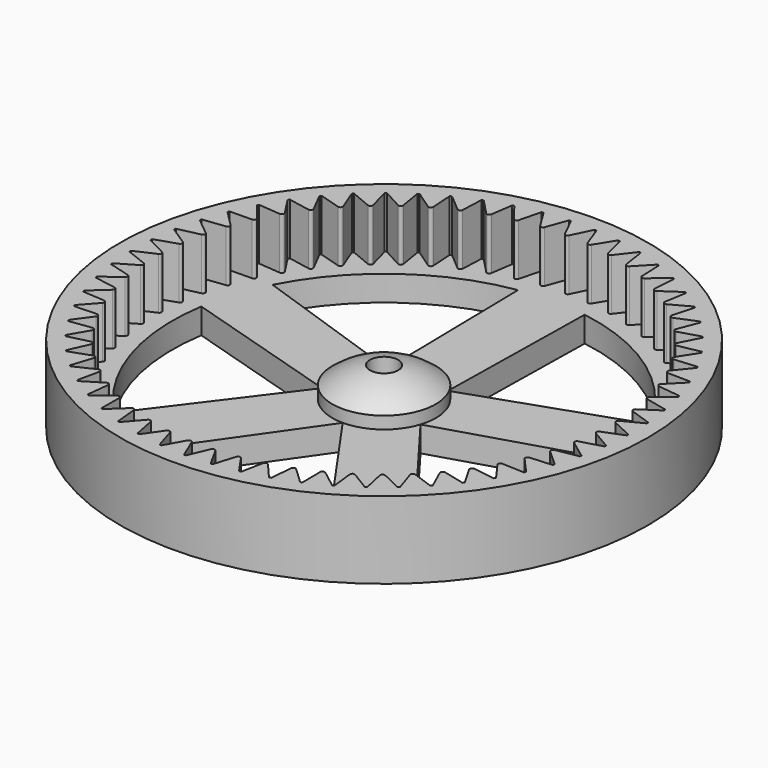
from build123d import *

# Parameters (mm, degrees)
F0_R            = 28.05
F1_DEPTH        = 2.7
F3_DEPTH        = 5.5
F3_COPIES_COUNT = 61
F2_R            = 28.05
F4_DEPTH        = 5.5
F8_DEPTH        = 2.7
F8_COPIES_COUNT = 5
F7_R            = 1.5
F9_DEPTH        = 1.5
F10_DEPTH       = 8.201


# Not quite as in the source:
# - a pattern or mirror of a feature is missing from the dataset's text; its kind, count and spacing are read off the source's solid
# - a feature names something its author has since deleted; it is built from what else it names


with BuildPart() as f1:
    # F0 (on Top) → F1 (new body)
    with BuildSketch(Plane.XY):
        Circle(F0_R)
    extrude(amount=F1_DEPTH)

    # F2 (on face) → F3 (join)
    with BuildSketch(Plane.XY.offset(2.7)):
        with BuildLine():
            ThreePointArc((-1.2632800726, 26.4198149777), (0, 26.45), (1.2632800726, 26.4198149777))
            Line((1.2632800726, 26.4198149777), (1.2934127659, 27.05))
            Line((1.2934127659, 27.05), (-1.2934127659, 27.05))
            Line((-1.2934127659, 27.05), (-1.2632800726, 26.4198149777))
        make_face()
        with BuildLine():
            Line((0.2246985116, 24.2904072133), (1.2632800726, 26.4198149777))
            ThreePointArc((1.2632800726, 26.4198149777), (0, 26.45), (-1.2632800726, 26.4198149777))
            Line((-1.2632800726, 26.4198149777), (-0.2246985116, 24.2904072133))
            ThreePointArc((-0.2246985116, 24.2904072133), (0, 24.15), (0.2246985116, 24.2904072133))
        make_face()
    f3 = extrude(amount=F3_DEPTH)

    # F3_copies: F3 ×61 about axis
    f3_copies_axis = Axis((0, 0, 0), (0, 0, 1))
    for i in range(1, F3_COPIES_COUNT):
        add(f3.rotate(f3_copies_axis, i * 360 / F3_COPIES_COUNT))

    # F2 (on face) → F4 (join, through all)
    with BuildSketch(Plane.XY.offset(2.7)):
        Circle(F2_R)
        with BuildLine():
            ThreePointArc((1.2632800726, 26.4198149777), (19.1444020267, 18.2508731583), (26.45, 0))
            ThreePointArc((26.45, 0), (-18.2508731583, -19.1444020267), (-1.2632800726, 26.4198149777))
            Line((-1.2632800726, 26.4198149777), (-1.2934127659, 27.05))
            Line((-1.2934127659, 27.05), (1.2934127659, 27.05))
            Line((1.2934127659, 27.05), (1.2632800726, 26.4198149777))
        make_face(mode=Mode.SUBTRACT)
    extrude(amount=F4_DEPTH)

    # F5 (on Front) → F6 (revolve)
    with BuildSketch(Plane.XZ):
        with BuildLine():
            Line((-5.5, 4), (-5.5, 0))
            Line((-5.5, 0), (0, 0))
            Line((0, 0), (0, 6))
            ThreePointArc((0, 6), (-2.9261749777, 5.4844811886), (-5.5, 4))
        make_face()
    revolve(axis=Axis((0, 0, 3), (0, 0, -1)))

    # F7 (on face) → F8 (cut, through all)
    with BuildSketch(Plane(origin=(0, 0, 0), x_dir=(1, 0, 0), z_dir=(0, 0, -1))):
        with BuildLine():
            Line((0, 5.5), (10.1938365841, 20.0583073986))
            ThreePointArc((10.1938365841, 20.0583073986), (0, 22.5), (-10.1938365841, 20.0583073986))
            Line((-10.1938365841, 20.0583073986), (0, 5.5))
        make_face()
    f8 = extrude(amount=-F8_DEPTH, mode=Mode.SUBTRACT)

    # F8_copies: F8 ×5 about axis
    f8_copies_axis = Axis((0, 0, 0), (0, 0, 1))
    for i in range(1, F8_COPIES_COUNT):
        add(f8.rotate(f8_copies_axis, i * 360 / F8_COPIES_COUNT), mode=Mode.SUBTRACT)

    # F7 (on face) → F9 (cut)
    with BuildSketch(Plane(origin=(0, 0, 0), x_dir=(1, 0, 0), z_dir=(0, 0, -1))):
        Polygon((1.7320508076, 3), (-1.7320508076, 3), (-3.4641016151, 0), (-1.7320508076, -3), (1.7320508076, -3), (3.4641016151, 0), align=None)
        Circle(F7_R, mode=Mode.SUBTRACT)
        Circle(F7_R)
    extrude(amount=-F9_DEPTH, mode=Mode.SUBTRACT)

    # F7 (on face) → F10 (cut, through all)
    with BuildSketch(Plane(origin=(0, 0, 0), x_dir=(1, 0, 0), z_dir=(0, 0, -1))):
        Circle(F7_R)
    extrude(amount=-F10_DEPTH, mode=Mode.SUBTRACT)


solid = f1.part
